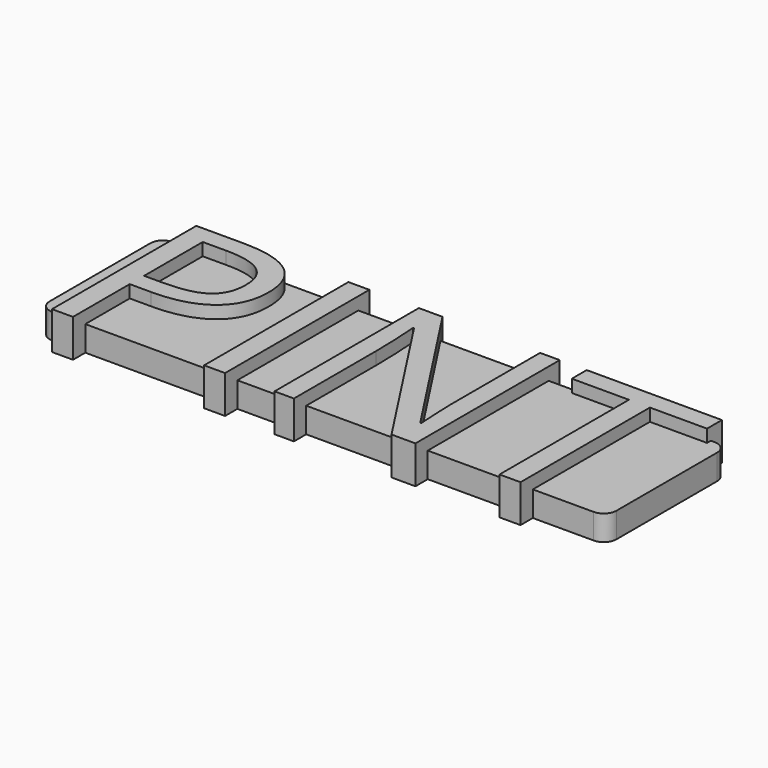
from build123d import *

# Parameters (mm, degrees)
F0_W          = 90
F0_H          = 24
F1_DEPTH      = 4
F2_R          = 2
F3_W          = 3.3284580025
F3_H          = 2.4421228583
F3_W_2        = 3.0777267029
F3_H_2        = 2.1976598412
F3_H_3        = 24
F3_W_3        = 3.1153363978
F3_W_4        = 21.4688675303
F4_DEPTH      = 2
F4_DEPTH_BACK = 4
F5_TEXT_SIZE  = 17.3611111111
F6_DEPTH      = 1.5


# Not quite as in the source:
# - a feature names something its author has since deleted; it is built from what else it names
# - Text() gives the source's letters only with a copy of the font that has no kerning and outlines rounded to 1/6400 em; it was checked with that copy


with BuildPart() as f1:
    # F0 (on Top) → F1 (new body)
    with BuildSketch(Plane.XY):
        Rectangle(F0_W, F0_H)
    extrude(amount=F1_DEPTH)

    # F2
    f2_edges = [f1.edges().sort_by_distance(p)[0] for p in [
        (-45, -12, 2),
        (45, 12, 2),
        (-45, 12, 2),
        (45, -12, 2),
    ]]
    fillet(f2_edges, radius=F2_R)

    # F3 (on face) → F4 (join, two sides)
    with BuildSketch(Plane.XY.offset(4)) as f4_sk:
        with Locations((-39.3992895947, -13.2210614292)):
            Rectangle(F3_W, F3_H)
        with BuildLine():
            add(Edge.make_bspline(
                [(-22.9043042206, 5.8545758462), (-22.9043042206, 1.5043877977), (-25.8723359799, -0.8368157125)],
                knots=[0, 0, 0, 1, 1, 1], degree=2))
            add(Edge.make_bspline(
                [(-25.4469719439, 12), (-22.9043042206, 9.9156905924), (-22.9043042206, 5.8545758462)],
                knots=[0.5132357832, 0.5132357832, 0.5132357832, 1, 1, 1], degree=2))
            Line((-25.4469719439, 12), (-41.0635185959, 12))
            Line((-41.0635185959, 12), (-41.0635185959, -12))
            Line((-41.0635185959, -12), (-37.7350605934, -12))
            Line((-37.7350605934, -12), (-37.7350605934, -3.1780192227))
            Line((-37.7350605934, -3.1780192227), (-34.3627246135, -3.1780192227))
            add(Edge.make_bspline(
                [(-25.8723359799, -0.8368157125), (-28.8403677392, -3.1780192227), (-34.3627246135, -3.1780192227)],
                knots=[0, 0, 0, 1, 1, 1], degree=2))
        make_face()
        with BuildLine():
            Line((-34.7325532804, -0.319682407), (-37.7350605934, -0.319682407))
            Line((-37.7350605934, -0.319682407), (-37.7350605934, 11.3142498955))
            Line((-37.7350605934, 11.3142498955), (-34.011700794, 11.3142498955))
            add(Edge.make_bspline(
                [(-28.2135394902, 9.9258253239), (-30.0752193899, 11.3142498955), (-34.011700794, 11.3142498955)],
                knots=[0, 0, 0, 1, 1, 1], degree=2))
            add(Edge.make_bspline(
                [(-26.3518595905, 5.697868784), (-26.3518595905, 8.5374007522), (-28.2135394902, 9.9258253239)],
                knots=[0, 0, 0, 1, 1, 1], degree=2))
            add(Edge.make_bspline(
                [(-28.3295027163, 1.1094860008), (-26.3518595905, 2.5386544087), (-26.3518595905, 5.697868784)],
                knots=[0, 0, 0, 1, 1, 1], degree=2))
            add(Edge.make_bspline(
                [(-34.7325532804, -0.319682407), (-30.307145842, -0.319682407), (-28.3295027163, 1.1094860008)],
                knots=[0, 0, 0, 1, 1, 1], degree=2))
        make_face(mode=Mode.SUBTRACT)
        Polygon((16.6422900125, -12), (11.253209838, -12), (12.8437108232, -14.4421228583), (16.6422900125, -14.4421228583), align=None)
        with Locations((-4.190346845, -13.2210614292)):
            Rectangle(F3_W_2, F3_H)
        with Locations((31.6642290013, -13.2210614292)):
            Rectangle(F3_W, F3_H)
        with BuildLine():
            Line((-41.0635185959, 12), (-25.4469719439, 12))
            add(Edge.make_bspline(
                [(-33.6356038445, 14.1976598412), (-28.1279168769, 14.1976598412), (-25.4469719439, 12)],
                knots=[0, 0, 0, 0.5132357832, 0.5132357832, 0.5132357832], degree=2))
            Line((-33.6356038445, 14.1976598412), (-41.0635185959, 14.1976598412))
            Line((-41.0635185959, 14.1976598412), (-41.0635185959, 12))
        make_face()
        with Locations((-15.2475971584, 13.0988299206)):
            Rectangle(F3_W, F3_H_2)
        with Locations((-15.2475971584, 0)):
            Rectangle(F3_W, F3_H_3)
        with Locations((-15.2475971584, -13.2210614292)):
            Rectangle(F3_W, F3_H)
        Polygon((-5.7292101964, 14.1976598412), (-5.7292101964, 12), (-0.5347841259, 12), (-1.968240702, 14.1976598412), align=None)
        with BuildLine():
            Line((-0.5347841259, 12), (-5.7292101964, 12))
            Line((-5.7292101964, 12), (-5.7292101964, -12))
            Line((-5.7292101964, -12), (-2.6514834935, -12))
            Line((-2.6514834935, -12), (-2.6514834935, 1.8366067697))
            add(Edge.make_bspline(
                [(-2.9648976181, 9.5904722106), (-2.6514834935, 5.3593815295), (-2.6514834935, 1.8366067697)],
                knots=[0, 0, 0, 1, 1, 1], degree=2))
            Line((-2.9648976181, 9.5904722106), (-2.8081905558, 9.5904722106))
            Line((-2.8081905558, 9.5904722106), (11.253209838, -12))
            Line((11.253209838, -12), (16.6422900125, -12))
            Line((16.6422900125, -12), (16.6422900125, 12))
            Line((16.6422900125, 12), (13.5269536147, 12))
            Line((13.5269536147, 12), (13.5269536147, -2.2377768491))
            add(Edge.make_bspline(
                [(13.6272461346, -6.3435018805), (13.4893439198, -3.4726284998), (13.5269536147, -2.2377768491)],
                knots=[0, 0, 0, 1, 1, 1], degree=2))
            add(Edge.make_bspline(
                [(13.8027580443, -9.7409109904), (13.7651483494, -9.2143752612), (13.6272461346, -6.3435018805)],
                knots=[0, 0, 0, 1, 1, 1], degree=2))
            Line((13.8027580443, -9.7409109904), (13.646050982, -9.7409109904))
            Line((13.646050982, -9.7409109904), (-0.5347841259, 12))
        make_face()
        with Locations((15.0846218136, 13.0988299206)):
            Rectangle(F3_W_3, F3_H_2)
        Polygon((42.3986627664, 12), (20.9297952361, 12), (20.9297952361, 11.2390305056), (30, 11.2390305056), (30, -12), (33.3284580025, -12), (33.3284580025, 11.2390305056), (42.3986627664, 11.2390305056), align=None)
        with Locations((31.6642290013, 13.0988299206)):
            Rectangle(F3_W_4, F3_H_2)
    extrude(amount=F4_DEPTH)
    extrude(f4_sk.sketch, amount=-F4_DEPTH_BACK)

    # F5 (on face) → F6 (cut)
    with BuildSketch(Plane(origin=(0, 0, 0), x_dir=(1, 0, 0), z_dir=(0, 0, -1))):
        with Locations((-26.3034396701, -6.25)):
            Text('4 cups', F5_TEXT_SIZE, font='Open Sans', text_align=(TextAlign.LEFT, TextAlign.BOTTOM))
    extrude(amount=-F6_DEPTH, mode=Mode.SUBTRACT)


solid = f1.part
